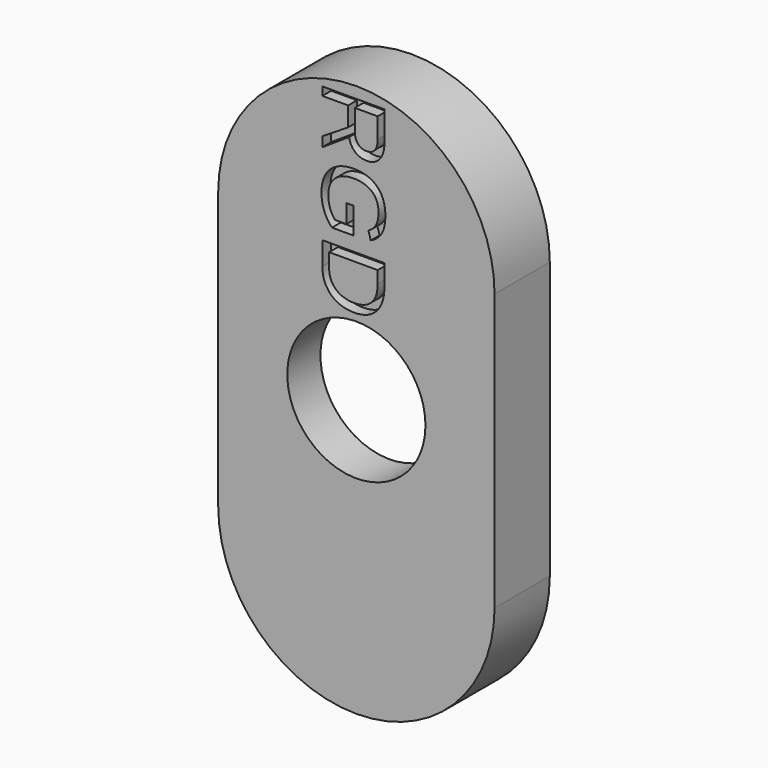
from build123d import *

# Parameters (mm, degrees)
F0_R         = 2.5
F1_DEPTH     = 1.5
F2_DEPTH     = 1
F3_TEXT_SIZE = 3.2660225639
F4_DEPTH     = 0.4


# Not quite as in the source:
# - Text() gives the source's letters only with a copy of the font that has no kerning and outlines rounded to 1/6400 em; it was checked with that copy


with BuildPart() as f1:
    # F0 (on Front) → F1 (new body)
    with BuildSketch(Plane.XZ):
        with BuildLine():
            ThreePointArc((0, -10), (3.5355339059, -8.5355339059), (5, -5))
            Line((5, -5), (5, 5))
            ThreePointArc((5, 5), (3.5355339059, 8.5355339059), (0, 10))
            ThreePointArc((0, 10), (-3.5355339059, 8.5355339059), (-5, 5))
            Line((-5, 5), (-5, -5))
            ThreePointArc((-5, -5), (-3.5355339059, -8.5355339059), (0, -10))
        make_face()
        with BuildLine():
            Line((3.5, 5), (3.5, -5))
            ThreePointArc((3.5, -5), (2.4748737342, -7.4748737342), (0, -8.5))
            ThreePointArc((0, -8.5), (-2.4748737342, -7.4748737342), (-3.5, -5))
            Line((-3.5, -5), (-3.5, 5))
            ThreePointArc((-3.5, 5), (-2.4748737342, 7.4748737342), (0, 8.5))
            ThreePointArc((0, 8.5), (2.4748737342, 7.4748737342), (3.5, 5))
        make_face(mode=Mode.SUBTRACT)
        with BuildLine():
            ThreePointArc((0, -8.5), (2.4748737342, -7.4748737342), (3.5, -5))
            Line((3.5, -5), (3.5, 5))
            ThreePointArc((3.5, 5), (2.4748737342, 7.4748737342), (0, 8.5))
            ThreePointArc((0, 8.5), (-2.4748737342, 7.4748737342), (-3.5, 5))
            Line((-3.5, 5), (-3.5, -5))
            ThreePointArc((-3.5, -5), (-2.4748737342, -7.4748737342), (0, -8.5))
        make_face()
        Circle(F0_R, mode=Mode.SUBTRACT)
    extrude(amount=F1_DEPTH)

    # F0 (on Front) → F2 (join)
    with BuildSketch(Plane.XZ):
        with BuildLine():
            ThreePointArc((0, -10), (3.5355339059, -8.5355339059), (5, -5))
            Line((5, -5), (5, 5))
            ThreePointArc((5, 5), (3.5355339059, 8.5355339059), (0, 10))
            ThreePointArc((0, 10), (-3.5355339059, 8.5355339059), (-5, 5))
            Line((-5, 5), (-5, -5))
            ThreePointArc((-5, -5), (-3.5355339059, -8.5355339059), (0, -10))
        make_face()
        with BuildLine():
            Line((3.5, 5), (3.5, -5))
            ThreePointArc((3.5, -5), (2.4748737342, -7.4748737342), (0, -8.5))
            ThreePointArc((0, -8.5), (-2.4748737342, -7.4748737342), (-3.5, -5))
            Line((-3.5, -5), (-3.5, 5))
            ThreePointArc((-3.5, 5), (-2.4748737342, 7.4748737342), (0, 8.5))
            ThreePointArc((0, 8.5), (2.4748737342, 7.4748737342), (3.5, 5))
        make_face(mode=Mode.SUBTRACT)
    extrude(amount=-F2_DEPTH)

    # F3 (on face) → F4 (cut)
    with BuildSketch(Plane.XZ.offset(1.5)):
        with Locations(Location((-1.2306325307, 9.8584180359), (0, 0, -90))):
            Text('RGD', F3_TEXT_SIZE, font='Arimo', text_align=(TextAlign.LEFT, TextAlign.BOTTOM))
    extrude(amount=-F4_DEPTH, mode=Mode.SUBTRACT)


solid = f1.part
